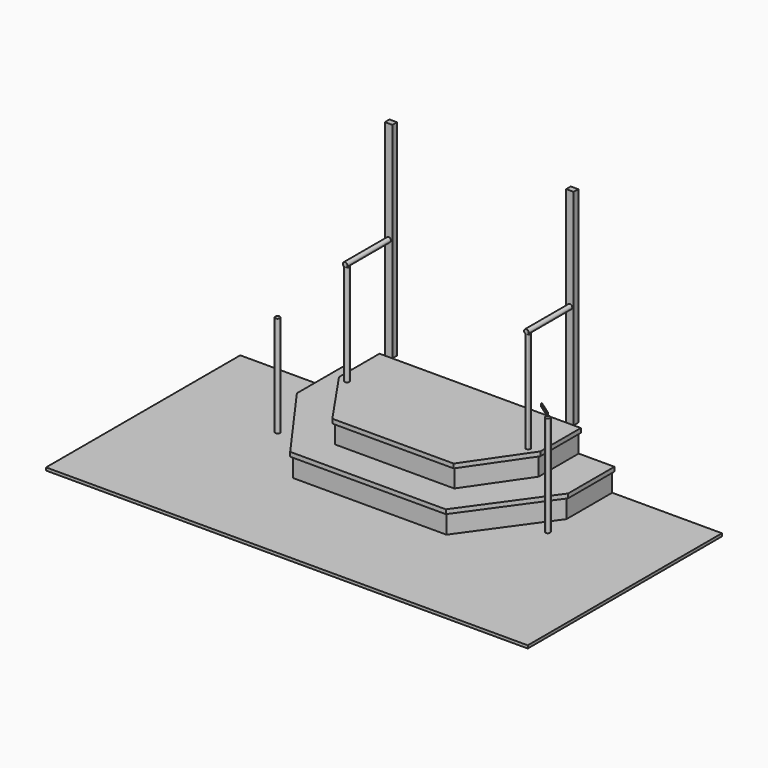
from build123d import *

# Parameters (mm, degrees)
F1_DEPTH  = 38.1
F3_DEPTH  = 168.275
F5_DEPTH  = 38.1
F7_DEPTH  = 171.45
F9_DEPTH  = 25.4
F10_W     = 66.675
F10_H     = 1828.8
F11_DEPTH = 50.8
F12_R     = 20.6375
F13_DEPTH = 898.525
F18_R     = 20.6375
F19_DEPTH = 898.525
F14_R     = 20.6375
F20_DEPTH = 484.1748
F21_R     = 20.6375
F23_DEPTH = 484.1748
F25_DEPTH = 25.4


# Not quite as in the source:
# - the program builds the solid bodies; features that only make, move or delete a surface that nothing else refers to are left out


with BuildPart() as f1:
    # F0 (on Top) → F1 (new body)
    with BuildSketch(Plane.XY):
        Polygon((0, -969.2605154219), (0, 0), (-895.35, 0), (-895.35, -450.85), (-539.75, -969.2605154219), align=None)
        Polygon((895.35, 0), (0, 0), (0, -969.2605154219), (539.75, -969.2605154219), (895.35, -450.85), align=None)
    extrude(amount=-F1_DEPTH)

    # F2 (on face) → F3 (join)
    with BuildSketch(Plane(origin=(0, 0, -38.1), x_dir=(1, 0, 0), z_dir=(0, 0, -1))):
        Polygon((-876.3, 0), (876.3, 0), (876.3, 444.9443133262), (529.7162480886, 950.2105154219), (-529.7162480886, 950.2105154219), (-876.3, 444.9443133262), align=None)
    extrude(amount=F3_DEPTH)

    # F4 (on face) → F5 (join)
    with BuildSketch(Plane(origin=(0, 0, -206.375), x_dir=(1, 0, 0), z_dir=(0, 0, -1))):
        Polygon((-1219.2, 0), (-876.3, 0), (-876.3, 444.9443133262), (-529.7162480886, 950.2105154219), (529.7162480886, 950.2105154219), (876.3, 444.9443133262), (876.3, 0), (1193.8, 0), (1193.8, 514.35), (679.45, 1231.6470793193), (-704.85, 1231.6470793193), (-1219.2, 514.35), align=None)
        Polygon((-876.3, 0), (0, 0), (876.3, 0), (876.3, 444.9443133262), (529.7162480886, 950.2105154219), (-529.7162480886, 950.2105154219), (-876.3, 444.9443133262), align=None)
    extrude(amount=F5_DEPTH)

    # F6 (on face) → F7 (join)
    with BuildSketch(Plane(origin=(0, 0, -244.475), x_dir=(1, 0, 0), z_dir=(0, 0, -1))):
        Polygon((1174.75, 0), (1174.75, 508.2258177526), (669.6686761911, 1212.5970793193), (-695.0686761911, 1212.5970793193), (-1200.15, 508.2258177526), (-1200.15, 0), align=None)
    extrude(amount=F7_DEPTH)

    # F12 (on face) → F13 (join)
    with BuildSketch(Plane.XY):
        with BuildLine():
            Line((798.5125, -463.55), (798.5125, -442.9125))
            ThreePointArc((798.5125, -442.9125), (780.2529386512, -473.1674230228), (815.5310270214, -475.2237373737))
            Line((815.5310270214, -475.2237373737), (798.5125, -463.55))
        make_face()
        with BuildLine():
            ThreePointArc((815.5310270214, -475.2237373737), (818.2245046882, -469.6609146143), (819.15, -463.55))
            ThreePointArc((819.15, -463.55), (813.1054161967, -448.9570838033), (798.5125, -442.9125))
            Line((798.5125, -442.9125), (798.5125, -463.55))
            Line((798.5125, -463.55), (815.5310270214, -475.2237373737))
        make_face()
        with Locations((-814.3748, -463.55)):
            Circle(F12_R)
    extrude(amount=F13_DEPTH)


with BuildPart() as f9:
    # F8 (on face) → F9 (new body)
    with BuildSketch(Plane(origin=(0, 0, -415.925), x_dir=(1, 0, 0), z_dir=(0, 0, -1))):
        Polygon((-2134.432844689, 0), (-1200.15, 0), (-1200.15, 508.2258177526), (-695.0686761911, 1212.5970793193), (0, 1212.5970793193), (0, 2159), (-2134.432844689, 2159), align=None)
        Polygon((0, 2159), (0, 1212.5970793193), (669.6686761911, 1212.5970793193), (1174.75, 508.2258177526), (1174.75, 0), (2150.4339796972, 0), (2150.4339796972, 2159), align=None)
    extrude(amount=F9_DEPTH)

    # F18 (on face) → F19 (join)
    with BuildSketch(Plane.XY.offset(-415.925)):
        with BuildLine():
            ThreePointArc((1214.4375, -740.3332872601), (1208.3929161967, -725.7403710633), (1193.8, -719.6957872601))
            Line((1193.8, -719.6957872601), (1193.8, -740.3332872601))
            Line((1193.8, -740.3332872601), (1210.705250314, -752.1704709653))
            ThreePointArc((1210.705250314, -752.1704709653), (1213.4823335711, -746.5391031973), (1214.4375, -740.3332872601))
        make_face()
        with BuildLine():
            ThreePointArc((1193.8, -719.6957872601), (1184.2706629944, -722.0276011904), (1176.894749686, -728.4961035549))
            Line((1176.894749686, -728.4961035549), (1193.8, -740.3332872601))
            Line((1193.8, -740.3332872601), (1193.8, -719.6957872601))
        make_face()
        with BuildLine():
            Line((1193.8, -740.3332872601), (1176.894749686, -728.4961035549))
            ThreePointArc((1176.894749686, -728.4961035549), (1175.4943139303, -749.8626242657), (1193.8, -760.9707872601))
            Line((1193.8, -760.9707872601), (1193.8, -740.3332872601))
        make_face()
        with BuildLine():
            Line((1210.705250314, -752.1704709653), (1193.8, -740.3332872601))
            Line((1193.8, -740.3332872601), (1193.8, -760.9707872601))
            ThreePointArc((1193.8, -760.9707872601), (1203.3293370056, -758.6389733298), (1210.705250314, -752.1704709653))
        make_face()
        with Locations((-1209.675, -740.3332872601)):
            Circle(F18_R)
    extrude(amount=F19_DEPTH)


with BuildPart() as f11:
    # F10 (on face) → F11 (new body)
    with BuildSketch(Plane(origin=(0, 0, 0), x_dir=(-1, 0, 0), z_dir=(0, 1, 0))):
        with Locations((814.3875, 914.4)):
            Rectangle(F10_W, F10_H)
    extrude(amount=F11_DEPTH)


with BuildPart() as f11b:
    # F10 (on face) → F11, piece 2 (new body)
    with BuildSketch(Plane(origin=(0, 0, 0), x_dir=(-1, 0, 0), z_dir=(0, 1, 0))):
        with Locations((-798.5125, 914.4)):
            Rectangle(F10_W, F10_H)
    extrude(amount=F11_DEPTH)


with BuildPart() as f20:
    # F14 (on face) → F20 (new body)
    with BuildSketch(Plane.XZ):
        with Locations((798.5125, 919.1625)):
            Circle(F14_R)
    extrude(amount=F20_DEPTH)


with BuildPart() as f23:
    # F21 (on face) → F23 (new body)
    with BuildSketch(Plane.XZ):
        with Locations((-814.3875, 919.1625)):
            Circle(F21_R)
    extrude(amount=F23_DEPTH)


with BuildPart() as f25:
    # F24 (on face) → F25 (new body)
    with BuildSketch(Plane.XY.offset(482.6)):
        with BuildLine():
            Line((1061.451881372, -638.8455143858), (1057.3094238, -644.7615569102))
            Line((1057.3094238, -644.7615569102), (1176.894749686, -728.4961035549))
            ThreePointArc((1176.894749686, -728.4961035549), (1179.2689059117, -725.6788097584), (1182.1061723691, -723.3285584593))
            Line((1182.1061723691, -723.3285584593), (1061.451881372, -638.8455143858))
        make_face()
    extrude(amount=F25_DEPTH)


solid = Compound([f1.part, f9.part, f11.part, f11b.part, f20.part, f23.part, f25.part])
